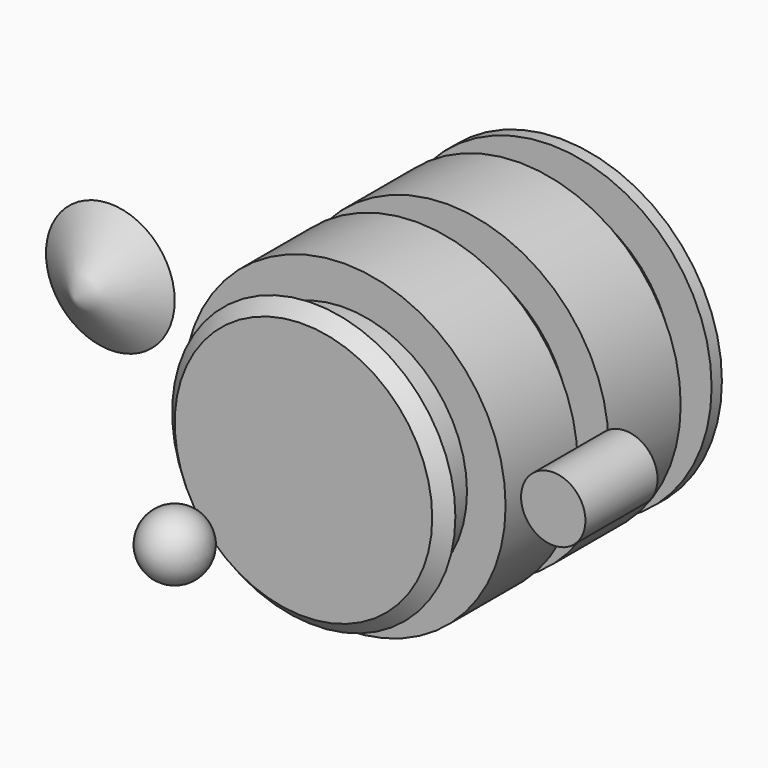
from build123d import *

# Parameters (mm, degrees)
F0_R     = 25
F1_DEPTH = 25
F5_R     = 5
F6_DEPTH = 14


# Not quite as in the source:
# - a fillet or chamfer that OpenCascade refuses, or shapes differently, is made with other operations: its cross-section is extruded or revolved along the edge and cut away or added


with BuildPart() as f1:
    # F0 (on Front) → F1 (new body, symmetric)
    with BuildSketch(Plane.XZ):
        Circle(F0_R)
    extrude(amount=F1_DEPTH, both=True)


with BuildPart() as f3:
    # F2 (on Top) → F3 (revolve)
    with BuildSketch(Plane.XY):
        Polygon((0, 25), (0, -25), (25, -25), (25, -23), (19, -23), (19, -17), (25, -17), (25, -3), (19, -3), (19, 3), (25, 3), (25, 17), (19, 17), (19, 23), (25, 23), (25, 25), align=None)
    revolve(axis=Axis((0, 0, 0), (0, 1, 0)))

    # F9: chamfer of 5 on 1 edges, made by hand

    # F9_s1 → F9_t2 (revolve, cut)
    with BuildSketch(Plane.XY):
        Polygon((20, -25), (25, -20), (25, -25), align=None)
    revolve(axis=Axis((0, -25, 0), (0, 1, 0)), mode=Mode.SUBTRACT)


with BuildPart() as f6:
    # F5 (on Front) → F6 (new body)
    with BuildSketch(Plane.XZ):
        with Locations((30, 0)):
            Circle(F5_R)
    extrude(amount=F6_DEPTH)


with BuildPart() as f8:
    # F7 (on Top) → F8 (revolve)
    with BuildSketch(Plane.XY):
        with BuildLine():
            ThreePointArc((0, -55), (5, -50), (0, -45))
            Line((0, -45), (0, -55))
        make_face()
    revolve(axis=Axis((0, -50, 0), (0, 1, 0)))


with BuildPart() as f11:
    # F10 (on Top) → F11 (revolve)
    with BuildSketch(Plane.XY):
        Polygon((-50, 7), (-50, 0), (-50, -7), (-40, 0), align=None)
    revolve(axis=Axis((-50, -3.5, 0), (0, -1, 0)))


solid = Compound([f3.part, f6.part, f8.part, f11.part])
